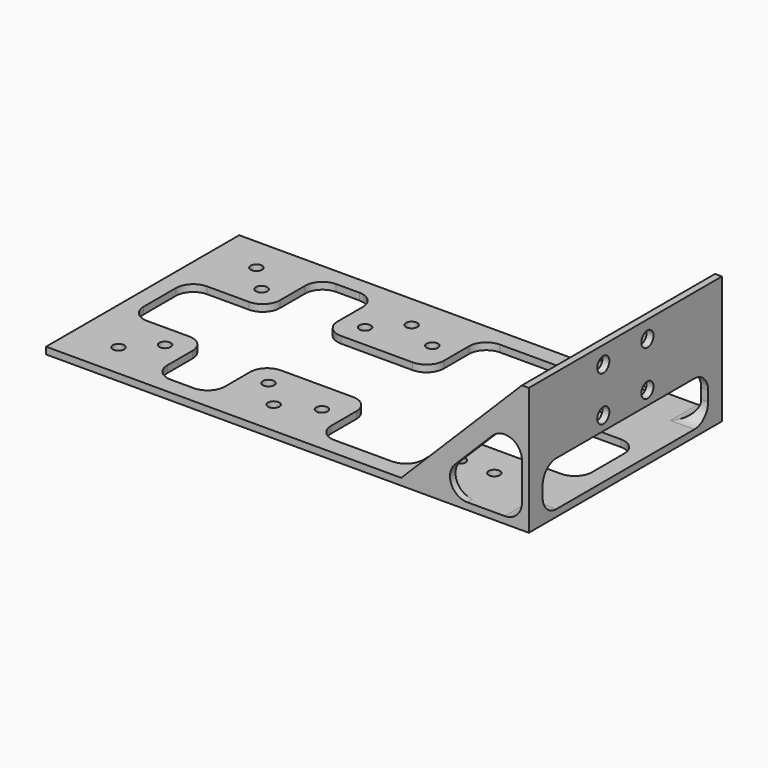
from build123d import *

# Parameters (mm, degrees)
F0_W      = 140
F0_H      = 70
F1_DEPTH  = 37
F2_W      = 138
F2_H      = 35
F3_DEPTH  = 70.001
F5_D      = 3.3
F6_W      = 2
F6_H      = 35
F7_DEPTH  = 35
F8_SIZE   = 34.99999
F10_DEPTH = 70.001
F11_W     = 60
F11_H     = 13
F12_DEPTH = 2.001
F13_W     = 33.65
F13_H     = 21.7
F13_W_2   = 26.7
F13_H_2   = 19.15
F13_W_3   = 30.8
F13_W_4   = 16.7
F13_W_5   = 22.15
F14_DEPTH = 2.001
F15_R     = 5
F17_D     = 4.4


# Not quite as in the source:
# - a fillet or chamfer is up to 0.001 mm smaller than in the source, because OpenCascade refuses the exact size
# - a feature names something its author has since deleted; it is built from what else it names


with BuildPart() as f1:
    # F0 (on Top) → F1 (new body)
    with BuildSketch(Plane.XY):
        with Locations((-10, 0)):
            Rectangle(F0_W, F0_H)
    extrude(amount=F1_DEPTH)

    # F2 (on face) → F3 (cut, through all)
    with BuildSketch(Plane.XZ.offset(35)):
        with Locations((-11, 19.5)):
            Rectangle(F2_W, F2_H)
    extrude(amount=-F3_DEPTH, mode=Mode.SUBTRACT)

    # F5 (through all)
    with Locations(Plane.XY.offset(2)):
        with Locations((-67, 25), (-59.5, 17.5), (-67, -25), (-59.5, -17.5), (-29.5, -17.5), (-22, -25), (-12, -20), (-12, 20), (-22, 25), (-29.5, 17.5), (28, 20), (38, 20), (38, -20), (28, -20)):
            Hole(F5_D / 2)

    # F6 (on face) → F7 (join)
    with BuildSketch(Plane(origin=(58, 0, 0), x_dir=(0, -1, 0), z_dir=(-1, 0, 0))):
        with Locations((-34, 19.5)):
            Rectangle(F6_W, F6_H)
        with Locations((34, 19.5)):
            Rectangle(F6_W, F6_H)
    extrude(amount=F7_DEPTH)

    # F8 (size 35 in the source; OpenCascade refuses exactly that, so slightly less here)
    f8_edges = [f1.edges().sort_by_distance(p)[0] for p in [
        (23, -34, 37),
        (23, 34, 37),
    ]]
    chamfer(f8_edges, length=F8_SIZE)

    # F9 (on face) → F10 (cut, through all)
    with BuildSketch(Plane.XZ.offset(35)):
        Polygon((58, 2), (58, 29.9289321881), (30.0710678119, 2), align=None)
    extrude(amount=-F10_DEPTH, mode=Mode.SUBTRACT)

    # F11 (on face) → F12 (cut, through all)
    with BuildSketch(Plane(origin=(58, 0, 0), x_dir=(0, -1, 0), z_dir=(-1, 0, 0))):
        with Locations((0, 8.5)):
            Rectangle(F11_W, F11_H)
    extrude(amount=-F12_DEPTH, mode=Mode.SUBTRACT)

    # F13 (on face) → F14 (cut, through all)
    with BuildSketch(Plane.XY.offset(2)):
        with Locations((38.175, 0)):
            Rectangle(F13_W, F13_H)
        with Locations((8, 0)):
            Rectangle(F13_W_2, F13_H)
        with Locations((8, 20.425)):
            Rectangle(F13_W_2, F13_H_2)
        with Locations((-20.75, 0)):
            Rectangle(F13_W_3, F13_H)
        with Locations((8, -20.425)):
            Rectangle(F13_W_2, F13_H_2)
        with Locations((-44.5, 0)):
            Rectangle(F13_W_4, F13_H)
        with Locations((-44.5, 20.425)):
            Rectangle(F13_W_4, F13_H_2)
        with Locations((-63.925, 0)):
            Rectangle(F13_W_5, F13_H)
        with Locations((-44.5, -20.425)):
            Rectangle(F13_W_4, F13_H_2)
    extrude(amount=-F14_DEPTH, mode=Mode.SUBTRACT)

    # F15 (call 1 of 28: OpenCascade refuses the feature's edges together)
    f15_edges = [f1.edges().sort_by_distance(p)[0] for p in [
        (55, 10.85, 1),
    ]]
    fillet(f15_edges, radius=F15_R)

    # F15#2 (call 2 of 28)
    f15_2_edges = [f1.edges().sort_by_distance(p)[0] for p in [
        (55, -10.85, 1),
    ]]
    fillet(f15_2_edges, radius=F15_R)

    # F15#3 (call 3 of 28)
    f15_3_edges = [f1.edges().sort_by_distance(p)[0] for p in [
        (21.35, -10.85, 1),
    ]]
    fillet(f15_3_edges, radius=F15_R)

    # F15#4 (call 4 of 28)
    f15_4_edges = [f1.edges().sort_by_distance(p)[0] for p in [
        (21.35, 10.85, 1),
    ]]
    fillet(f15_4_edges, radius=F15_R)

    # F15#5 (call 5 of 28)
    f15_5_edges = [f1.edges().sort_by_distance(p)[0] for p in [
        (21.35, -30, 1),
    ]]
    fillet(f15_5_edges, radius=F15_R)

    # F15#6 (call 6 of 28)
    f15_6_edges = [f1.edges().sort_by_distance(p)[0] for p in [
        (21.35, 30, 1),
    ]]
    fillet(f15_6_edges, radius=F15_R)

    # F15#7 (call 7 of 28)
    f15_7_edges = [f1.edges().sort_by_distance(p)[0] for p in [
        (-5.35, -30, 1),
    ]]
    fillet(f15_7_edges, radius=F15_R)

    # F15#8 (call 8 of 28)
    f15_8_edges = [f1.edges().sort_by_distance(p)[0] for p in [
        (-5.35, -10.85, 1),
    ]]
    fillet(f15_8_edges, radius=F15_R)

    # F15#9 (call 9 of 28)
    f15_9_edges = [f1.edges().sort_by_distance(p)[0] for p in [
        (-5.35, 10.85, 1),
    ]]
    fillet(f15_9_edges, radius=F15_R)

    # F15#10 (call 10 of 28)
    f15_10_edges = [f1.edges().sort_by_distance(p)[0] for p in [
        (-5.35, 30, 1),
    ]]
    fillet(f15_10_edges, radius=F15_R)

    # F15#11 (call 11 of 28)
    f15_11_edges = [f1.edges().sort_by_distance(p)[0] for p in [
        (-36.15, 10.85, 1),
    ]]
    fillet(f15_11_edges, radius=F15_R)

    # F15#12 (call 12 of 28)
    f15_12_edges = [f1.edges().sort_by_distance(p)[0] for p in [
        (-36.15, -30, 1),
    ]]
    fillet(f15_12_edges, radius=F15_R)

    # F15#13 (call 13 of 28)
    f15_13_edges = [f1.edges().sort_by_distance(p)[0] for p in [
        (-36.15, -10.85, 1),
    ]]
    fillet(f15_13_edges, radius=F15_R)

    # F15#14 (call 14 of 28)
    f15_14_edges = [f1.edges().sort_by_distance(p)[0] for p in [
        (-36.15, 30, 1),
    ]]
    fillet(f15_14_edges, radius=F15_R)

    # F15#15 (call 15 of 28)
    f15_15_edges = [f1.edges().sort_by_distance(p)[0] for p in [
        (-52.85, -30, 1),
    ]]
    fillet(f15_15_edges, radius=F15_R)

    # F15#16 (call 16 of 28)
    f15_16_edges = [f1.edges().sort_by_distance(p)[0] for p in [
        (-52.85, -10.85, 1),
    ]]
    fillet(f15_16_edges, radius=F15_R)

    # F15#17 (call 17 of 28)
    f15_17_edges = [f1.edges().sort_by_distance(p)[0] for p in [
        (-75, -10.85, 1),
    ]]
    fillet(f15_17_edges, radius=F15_R)

    # F15#18 (call 18 of 28)
    f15_18_edges = [f1.edges().sort_by_distance(p)[0] for p in [
        (-52.85, 10.85, 1),
    ]]
    fillet(f15_18_edges, radius=F15_R)

    # F15#19 (call 19 of 28)
    f15_19_edges = [f1.edges().sort_by_distance(p)[0] for p in [
        (-75, 10.85, 1),
    ]]
    fillet(f15_19_edges, radius=F15_R)

    # F15#20 (call 20 of 28)
    f15_20_edges = [f1.edges().sort_by_distance(p)[0] for p in [
        (-52.85, 30, 1),
    ]]
    fillet(f15_20_edges, radius=F15_R)

    # F15#21 (call 21 of 28)
    f15_21_edges = [f1.edges().sort_by_distance(p)[0] for p in [
        (30.071068, -34, 2),
    ]]
    fillet(f15_21_edges, radius=F15_R)

    # F15#22 (call 22 of 28)
    f15_22_edges = [f1.edges().sort_by_distance(p)[0] for p in [
        (30.071068, 34, 2),
    ]]
    fillet(f15_22_edges, radius=F15_R)

    # F15#23 (call 23 of 28)
    f15_23_edges = [f1.edges().sort_by_distance(p)[0] for p in [
        (58, 32.5, 2),
        (59, 30, 2),
    ]]
    fillet(f15_23_edges, radius=F15_R)

    # F15#24 (call 24 of 28)
    f15_24_edges = [f1.edges().sort_by_distance(p)[0] for p in [
        (58, 34, 29.928932),
    ]]
    fillet(f15_24_edges, radius=F15_R)

    # F15#25 (call 25 of 28)
    f15_25_edges = [f1.edges().sort_by_distance(p)[0] for p in [
        (58, -32.5, 2),
        (59, -30, 2),
    ]]
    fillet(f15_25_edges, radius=F15_R)

    # F15#26 (call 26 of 28)
    f15_26_edges = [f1.edges().sort_by_distance(p)[0] for p in [
        (58, -34, 29.928932),
    ]]
    fillet(f15_26_edges, radius=F15_R)

    # F15#27 (call 27 of 28)
    f15_27_edges = [f1.edges().sort_by_distance(p)[0] for p in [
        (59, -30, 15),
    ]]
    fillet(f15_27_edges, radius=F15_R)

    # F15#28 (call 28 of 28)
    f15_28_edges = [f1.edges().sort_by_distance(p)[0] for p in [
        (59, 30, 15),
    ]]
    fillet(f15_28_edges, radius=F15_R)

    # F17 (through all)
    with Locations(Plane.YZ.offset(60)):
        with Locations((-8, 32), (8, 32), (-8, 19), (8, 19)):
            Hole(F17_D / 2)


solid = f1.part
